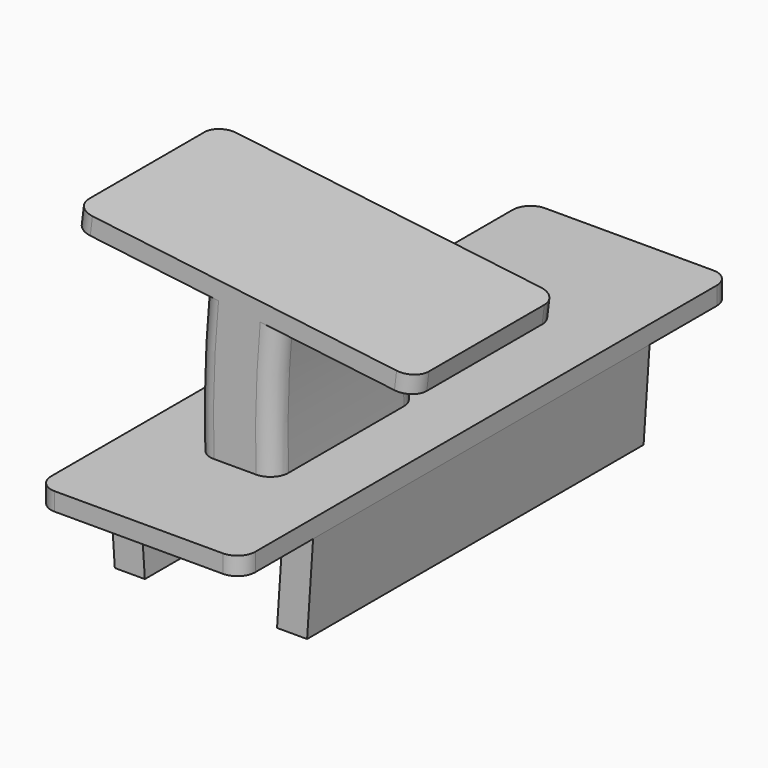
from build123d import *

# Parameters (mm, degrees)
F0_W     = 34
F0_H     = 102
F1_DEPTH = 3
F6_W     = 57
F6_H     = 30
F7_DEPTH = 3
F8_R     = 3
F2_W     = 5
F2_H     = 70
F10_W    = 5
F10_H    = 70
F13_R    = 3


# Not quite as in the source:
# - a feature names something its author has since deleted; it is built from what else it names


with BuildPart() as f1:
    # F0 (on Top) → F1 (new body)
    with BuildSketch(Plane.XY):
        with Locations((0, 1)):
            Rectangle(F0_W, F0_H)
    extrude(amount=F1_DEPTH)

    # F5: sweep along a path in F4
    with BuildLine(Plane.XZ) as f5_path:
        ThreePointArc((0.7317709574, 26), (0.0173632461, 14.5110886282), (0, 3))
    # F3 (on face) → F5 (sweep)
    with BuildSketch(Plane.XY.offset(3)):
        Polygon((6.5, 0), (0, 0), (-6.5, 0), (-6.5, -30), (0, -30), (6.5, -30), align=None)
    sweep(path=f5_path.line)

    # F6 (on face) → F7 (join)
    with BuildSketch(Plane(origin=(3.1308235326, 0, 25.7078318269), x_dir=(0.9926657135, 0, -0.1208916099), z_dir=(0.1208916099, 0, 0.9926657135))):
        with Locations((-1.916777917, -15)):
            Rectangle(F6_W, F6_H)
    extrude(amount=F7_DEPTH)

    # F8
    f8_edges = [f1.edges().sort_by_distance(p)[0] for p in [
        (29.700414, -30, 23.983142),
        (29.700414, 0, 23.983142),
        (-26.881532, -30, 30.873964),
        (-26.881532, 0, 30.873964),
    ]]
    fillet(f8_edges, radius=F8_R)

    # F2 (on face) → F11 section 0
    with BuildSketch(Plane(origin=(0, 0, 0), x_dir=(1, 0, 0), z_dir=(0, 0, -1))):
        with Locations((14.5, 0)):
            Rectangle(F2_W, F2_H)
    # F10 (on offset) → F11 section 1
    with BuildSketch(Plane.XY.offset(-15)):
        with Locations((13.5, 0)):
            Rectangle(F10_W, F10_H)
    loft()

    # F2 (on face) → F12 section 0
    with BuildSketch(Plane(origin=(0, 0, 0), x_dir=(1, 0, 0), z_dir=(0, 0, -1))):
        with Locations((-14.5, 0)):
            Rectangle(F2_W, F2_H)
    # F10 (on offset) → F12 section 1
    with BuildSketch(Plane.XY.offset(-15)):
        with Locations((-13.5, 0)):
            Rectangle(F10_W, F10_H)
    loft()

    # F13
    f13_edges = [f1.edges().sort_by_distance(p)[0] for p in [
        (17, -50, 1.5),
        (-17, -50, 1.5),
        (17, 52, 1.5),
        (-17, 52, 1.5),
        (6.505434, -30, 14.117469),
        (-6.470708, -30, 14.904709),
        (6.505434, 0, 14.117469),
        (-6.470708, 0, 14.904709),
    ]]
    fillet(f13_edges, radius=F13_R)


solid = f1.part
